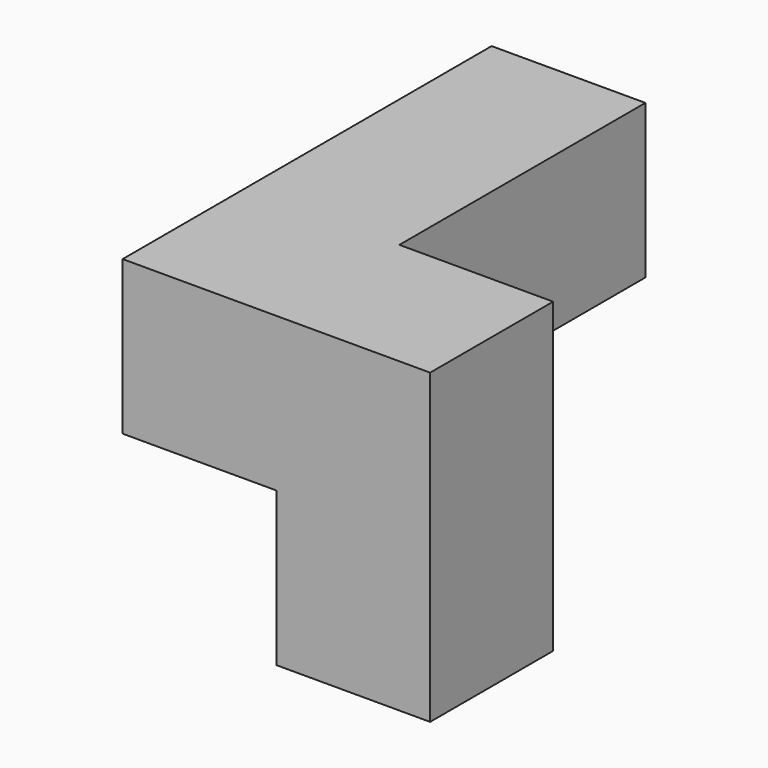
from build123d import *

# Parameters (mm, degrees)
F1_W     = 127
F1_H     = 127
F2_DEPTH = 190.5
F3_W     = 127
F3_H     = 127
F4_DEPTH = 127
F5_W     = 127
F5_H     = 127
F6_DEPTH = 127


# Not quite as in the source:
# - a variable given as a bare number and used for a length is read in inches; the dataset says mm whatever the document's units were


with BuildPart() as f2:
    # F1 (on Front) → F2 (new body, symmetric)
    with BuildSketch(Plane.XZ):
        Rectangle(F1_W, F1_H)
    extrude(amount=F2_DEPTH, both=True)

    # F3 (on face) → F4 (join)
    with BuildSketch(Plane.YZ.offset(63.5)):
        with Locations((-127, 0)):
            Rectangle(F3_W, F3_H)
    extrude(amount=F4_DEPTH)

    # F5 (on face) → F6 (join)
    with BuildSketch(Plane(origin=(0, 0, -63.5), x_dir=(1, 0, 0), z_dir=(0, 0, -1))):
        with Locations((127, 127)):
            Rectangle(F5_W, F5_H)
    extrude(amount=F6_DEPTH)


solid = f2.part
